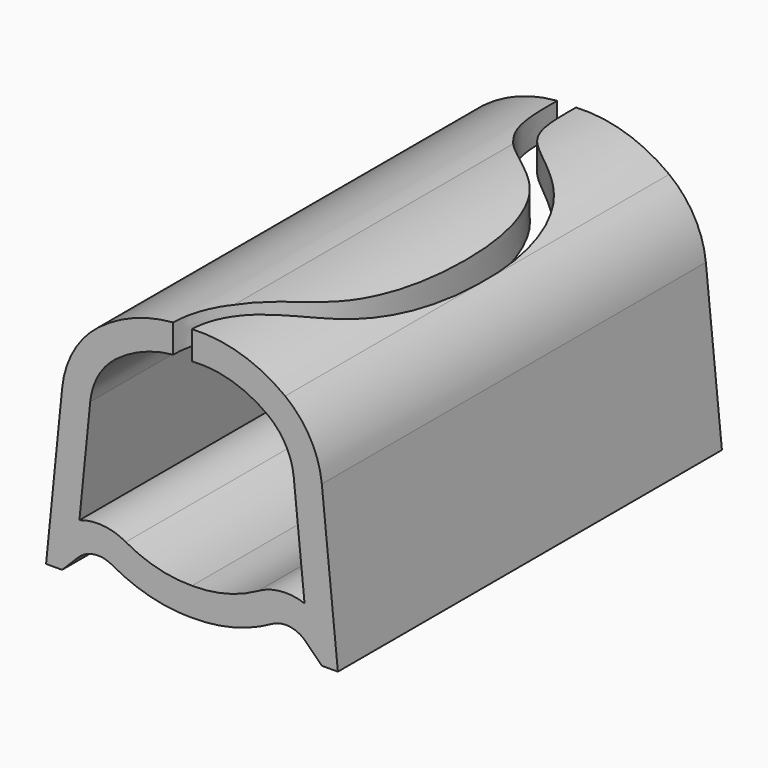
from build123d import *

# Parameters (mm, degrees)
F1_DEPTH = 2.55
F3_DEPTH = 25
F5_DEPTH = 25


# Not quite as in the source:
# - the dataset's text gives a spline's control points without its knots; the knots are read off the source's solid


with BuildPart() as f1:
    # F0 (on Front) → F1 (new body, symmetric)
    with BuildSketch(Plane.XZ):
        with BuildLine():
            Line((-1.3794310575, 0.35), (-1.55, -1.35))
            Line((-1.55, -1.35), (-1.38, -1.35))
            Line((-1.38, -1.35), (-1.21, -1.18))
            ThreePointArc((-1.21, -1.18), (-1.0385273379, -1.0949001124), (-0.8504995958, -1.1308227089))
            ThreePointArc((-0.8504995958, -1.1308227089), (-0.4396486045, -1.2962847488), (0, -1.35))
            ThreePointArc((0, -1.35), (0.4396486045, -1.2962847488), (0.8504995958, -1.1308227089))
            ThreePointArc((0.8504995958, -1.1308227089), (1.0385273379, -1.0949001124), (1.21, -1.18))
            Line((1.21, -1.18), (1.38, -1.35))
            Line((1.38, -1.35), (1.55, -1.35))
            Line((1.55, -1.35), (1.3794310575, 0.35))
            ThreePointArc((1.3794310575, 0.35), (1.2570591939, 0.7385443736), (0.9898813272, 1.0460465537))
            ThreePointArc((0.9898813272, 1.0460465537), (0.5220007527, 1.2861495252), (0, 1.35))
            ThreePointArc((0, 1.35), (-0.5220007527, 1.2861495252), (-0.9898813272, 1.0460465537))
            ThreePointArc((-0.9898813272, 1.0460465537), (-1.2570591939, 0.7385443736), (-1.3794310575, 0.35))
        make_face()
    extrude(amount=F1_DEPTH, both=True)

    # F2 (on face) → F3 (cut)
    with BuildSketch(Plane.XZ.offset(2.55)):
        with BuildLine():
            ThreePointArc((-1.1958934952, -0.825752383), (-0.9447923506, -0.7944841457), (-0.7031312179, -0.8695133691))
            ThreePointArc((-0.7031312179, -0.8695133691), (-0.3634662432, -1.0061149648), (0, -1.0499850117))
            ThreePointArc((0, -1.0499850117), (0.3634662432, -1.0061149648), (0.7031312179, -0.8695133691))
            ThreePointArc((0.7031312179, -0.8695133691), (0.9447923506, -0.7944841457), (1.1958934952, -0.825752383))
            Line((1.1958934952, -0.825752383), (1.0809297915, 0.3200499734))
            ThreePointArc((1.0809297915, 0.3200499734), (0.995269489, 0.5920310285), (0.8082449867, 0.8072825495))
            ThreePointArc((0.8082449867, 0.8072825495), (0.4261075642, 1.0017409157), (0, 1.0494421693))
            ThreePointArc((0, 1.0494421693), (-0.4261075642, 1.0017409157), (-0.8082449867, 0.8072825495))
            ThreePointArc((-0.8082449867, 0.8072825495), (-0.995269489, 0.5920310285), (-1.0809297915, 0.3200499734))
            Line((-1.0809297915, 0.3200499734), (-1.1958934952, -0.825752383))
        make_face()
    extrude(amount=-F3_DEPTH, mode=Mode.SUBTRACT)

    # F4 (on Top) → F5 (cut)
    with BuildSketch(Plane.XY):
        with BuildLine():
            add(Edge.make_bspline(
                [(0, 2.55), (0, 2.3012170484), (-0.0174660225, 1.8063678705), (0.8981223952, 1.4759598818), (1.0546660634, -0.0192739265), (0.8408673454, -1.4725471105), (0.1636337962, -2.021288105), (0, -2.3857110462), (0, -2.55)],
                knots=[0, 0, 0, 0, 0.1425106556, 0.297117234, 0.5049568696, 0.7167103753, 0.8747727514, 1, 1, 1, 1], degree=3))
            Line((0, 2.55), (-0.199999971, 2.55))
            add(Edge.make_bspline(
                [(-0.199999971, 2.55), (-0.199999971, 2.442861913), (-0.2033495667, 2.2756171701), (-0.1723667571, 2.0458653132), (-0.1168215656, 1.8712862158), (-0.0022501698, 1.7056297023), (0.1335578991, 1.590875413), (0.2688325655, 1.4955434762), (0.39494662, 1.4058304378), (0.5020185664, 1.3121894563), (0.6095184956, 1.1758498184), (0.7160601321, 0.9149098947), (0.781329804, 0.5035285403), (0.7939401967, 0.0406520803), (0.7709571004, -0.4234581557), (0.7074148963, -0.8510847156), (0.598032004, -1.2186029446), (0.4450309549, -1.4850813091), (0.2412797275, -1.7118129344), (0.0210326126, -1.9446414735), (-0.1511521088, -2.2249054182), (-0.199999971, -2.4387055988), (-0.199999971, -2.55)],
                knots=[0, 0, 0, 0, 0.0625, 0.09375, 0.125, 0.15625, 0.1875, 0.21875, 0.25, 0.28125, 0.3125, 0.375, 0.4375, 0.5, 0.5625, 0.625, 0.6875, 0.75, 0.8125, 0.875, 0.9375, 1, 1, 1, 1], degree=3))
            Line((-0.199999971, -2.55), (0, -2.55))
        make_face()
    extrude(amount=F5_DEPTH, mode=Mode.SUBTRACT)


solid = f1.part
